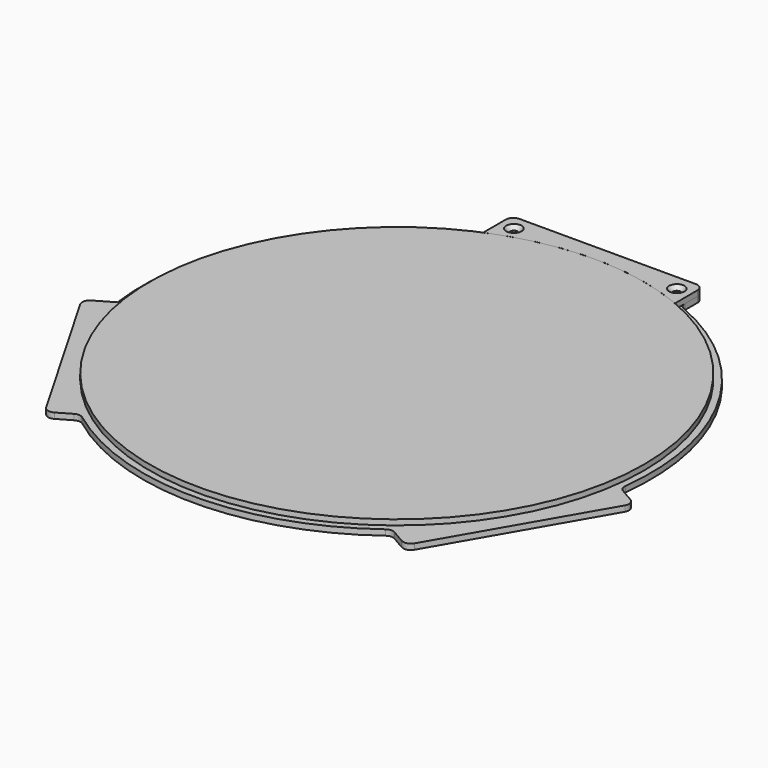
from build123d import *

# Parameters (mm, degrees)
F2_DEPTH       = 2.95
F3_D           = 3.2
F4_R           = 129
F5_DEPTH       = 2.8
F6_R           = 1.6
F7_DEPTH       = 2.8
F9_D           = 4
F9_CSINK_D     = 8
F9_CSINK_ANGLE = 90


# Not quite as in the source:
# - a feature names something its author has since deleted; it is built from what else it names


with BuildPart() as f2:
    # F1 (on Top) → F2 (new body)
    with BuildSketch(Plane.XY):
        with BuildLine():
            ThreePointArc((-83.5688145832, -105.9835045144), (-81.3352017208, -105.4544338279), (-79.1785196504, -106.2403502723))
            ThreePointArc((-79.1785196504, -106.2403502723), (0, -132.5), (79.1785196504, -106.2403502723))
            ThreePointArc((79.1785196504, -106.2403502723), (81.3352017208, -105.4544338279), (83.5688145832, -105.9835045144))
            Line((83.5688145832, -105.9835045144), (90.6143914052, -110.0512701892))
            ThreePointArc((90.6143914052, -110.0512701892), (93.6496675856, -110.4508718792), (96.0784930204, -108.5871685741))
            Line((96.0784930204, -108.5871685741), (142.0784930204, -28.9128314259))
            ThreePointArc((142.0784930204, -28.9128314259), (142.4780947104, -25.8775552455), (140.6143914052, -23.4487298108))
            Line((140.6143914052, -23.4487298108), (133.5688145832, -19.380964136))
            ThreePointArc((133.5688145832, -19.380964136), (131.9938194971, -17.7111339982), (131.5961020679, -15.4504343151))
            ThreePointArc((131.5961020679, -15.4504343151), (114.7483660014, 66.25), (52.4175824176, 121.6907845874))
            ThreePointArc((52.4175824176, 121.6907845874), (50.6586177763, 123.1655678261), (50, 125.3644686504))
            Line((50, 125.3644686504), (50, 133.5))
            ThreePointArc((50, 133.5), (48.8284271247, 136.3284271247), (46, 137.5))
            Line((46, 137.5), (-46, 137.5))
            ThreePointArc((-46, 137.5), (-48.8284271247, 136.3284271247), (-50, 133.5))
            Line((-50, 133.5), (-50, 125.3644686504))
            ThreePointArc((-50, 125.3644686504), (-50.6586177763, 123.1655678261), (-52.4175824176, 121.6907845874))
            ThreePointArc((-52.4175824176, 121.6907845874), (-115.3980732063, 65.1117093946), (-131.2647048648, -18.0506857698))
            Line((-131.2647048648, -18.0506857698), (-140.6143914052, -23.4487298108))
            ThreePointArc((-140.6143914052, -23.4487298108), (-142.4780947104, -25.8775552455), (-142.0784930204, -28.9128314259))
            Line((-142.0784930204, -28.9128314259), (-96.0784930204, -108.5871685741))
            ThreePointArc((-96.0784930204, -108.5871685741), (-93.6496675856, -110.4508718792), (-90.6143914052, -110.0512701892))
            Line((-90.6143914052, -110.0512701892), (-83.5688145832, -105.9835045144))
        make_face()
    extrude(amount=F2_DEPTH)

    # F3 (through all)
    with Locations(Plane(origin=(0, 0, 0), x_dir=(1, 0, 0), z_dir=(0, 0, -1))):
        with Locations((-42.5, -129.5), (42.5, -129.5)):
            Hole(F3_D / 2)


with BuildPart() as f5:
    # F4 (on face) → F5 (new body)
    with BuildSketch(Plane.XY.offset(2.95)):
        Circle(F4_R)
    extrude(amount=F5_DEPTH)


with BuildPart() as f7:
    # F6 (on face) → F7 (new body)
    with BuildSketch(Plane.XY.offset(2.95)):
        with BuildLine():
            ThreePointArc((-46, 137.5), (-48.8284271247, 136.3284271247), (-50, 133.5))
            Line((-50, 133.5), (-50, 125.3644686504))
            Line((-50, 125.3644686504), (-50, 118.9159366948))
            ThreePointArc((-50, 118.9159366948), (0, 129), (50, 118.9159366948))
            Line((50, 118.9159366948), (50, 125.3644686504))
            Line((50, 125.3644686504), (50, 133.5))
            ThreePointArc((50, 133.5), (48.8284271247, 136.3284271247), (46, 137.5))
            Line((46, 137.5), (-46, 137.5))
        make_face()
        with Locations((-42.5, 129.5)):
            Circle(F6_R, mode=Mode.SUBTRACT)
        with Locations((42.5, 129.5)):
            Circle(F6_R, mode=Mode.SUBTRACT)
    extrude(amount=F7_DEPTH)

    # F9 (through all)
    with Locations(Plane.XY.offset(5.75)):
        with Locations((42.5, 129.5), (-42.5, 129.5)):
            CounterSinkHole(F9_D / 2, F9_CSINK_D / 2, counter_sink_angle=F9_CSINK_ANGLE)


solid = Compound([f2.part, f5.part, f7.part])
